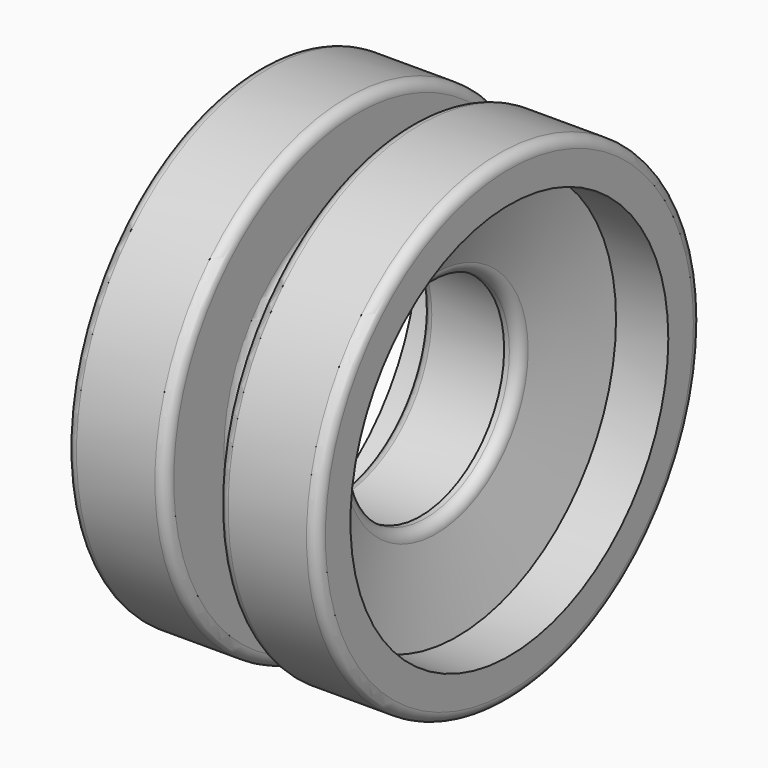
from build123d import *

# Parameters (mm, degrees)
F0_W = 1.5
F0_H = 1
F2_R = 0.99999


# Not quite as in the source:
# - a fillet or chamfer is up to 0.001 mm smaller than in the source, because OpenCascade refuses the exact size


with BuildPart() as f1:
    # F0 (on Top) → F1 (revolve)
    with BuildSketch(Plane.XY):
        Polygon((-12, 23), (-12, 19), (-7, 19), (-5, 11), (3.5, 11), (5, 11), (7, 19), (12, 19), (12, 23), (2.5, 23), (2.5, 15), (-2.5, 15), (-2.5, 23), align=None)
        with Locations((4.25, 10.5)):
            Rectangle(F0_W, F0_H)
    revolve(axis=Axis((0, 0, 0), (1, 0, 0)))

    # F2 (radius 1 in the source; OpenCascade refuses exactly that, so slightly less here)
    f2_edges = [f1.edges().sort_by_distance(p)[0] for p in [
        (-12, -23, 0),
        (-2.5, -23, 0),
        (2.5, -23, 0),
        (12, -23, 0),
        (2.5, -15, 0),
        (-2.5, -15, 0),
        (-5, -11, 0),
        (5, -10, 0),
    ]]
    fillet(f2_edges, radius=F2_R)


solid = f1.part
